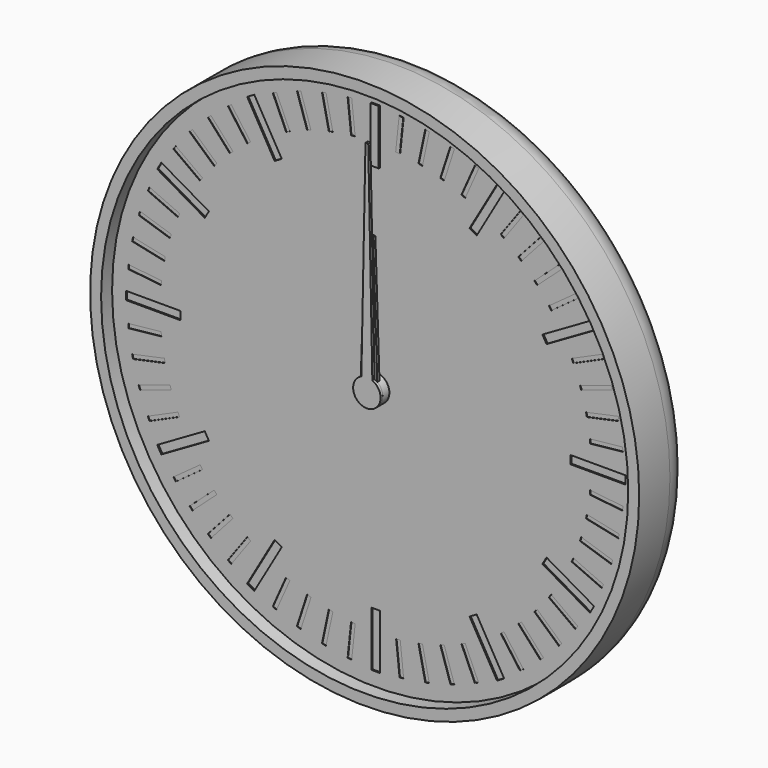
from build123d import *

# Parameters (mm, degrees)
F0_R      = 100
F1_DEPTH  = 24
F2_R      = 10
F3_T      = -4
F4_R      = 5
F4_R_2    = 3
F5_DEPTH  = 2
F6_DEPTH  = 19
F7_DEPTH  = 8
F9_DEPTH  = 4
F11_DEPTH = 4
F12_R     = 5
F12_R_2   = 3
F13_DEPTH = 2
F14_R     = 3
F15_DEPTH = 4
F17_DEPTH = 4
F18_R     = 3
F19_DEPTH = 2
F20_R     = 98
F20_R_2   = 5
F21_DEPTH = 1
F23_R     = 5
F23_R_2   = 3
F24_DEPTH = 2
F25_W     = 3
F25_H     = 20
F25_W_2   = 20
F25_H_2   = 3
F26_DEPTH = 0.5
F27_W     = 1.5
F27_H     = 12
F27_W_2   = 12
F27_H_2   = 1.5
F28_DEPTH = 0.2
F29_DEPTH = 1
F30_DEPTH = 0.4
F31_R     = 5
F31_R_2   = 3
F32_DEPTH = 5
F33_R     = 3
F34_DEPTH = 1
F36_DEPTH = 1


with BuildPart() as f1:
    # F0 (on Front) → F1 (new body)
    with BuildSketch(Plane.XZ):
        Circle(F0_R)
    extrude(amount=F1_DEPTH)

    # F2
    f2_edges = [f1.edges().sort_by_distance(p)[0] for p in [
        (-100, 0, 0),
    ]]
    fillet(f2_edges, radius=F2_R)

    # F3
    f3_openings = [f1.faces().sort_by_distance(p)[0] for p in [
        (0, -24, 0),
    ]]
    offset(amount=F3_T, openings=f3_openings)

    # F4 (on face) → F5 (join)
    with BuildSketch(Plane.XZ.offset(4)):
        Circle(F4_R)
        Circle(F4_R_2, mode=Mode.SUBTRACT)
        with Locations((40, 0)):
            Circle(F4_R)
        with Locations((40, 0)):
            Circle(F4_R_2, mode=Mode.SUBTRACT)
    extrude(amount=F5_DEPTH)


with BuildPart() as f6:
    # F6 (new): a face of the model
    f6_faces = [f1.part.faces().sort_by_distance(p)[0] for p in [
        (0, -4, 0),
    ]]
    extrude(f6_faces, amount=F6_DEPTH)

    # F8 (on face) → F9 (join)
    with BuildSketch(Plane.XZ.offset(6)):
        with BuildLine():
            ThreePointArc((9.2729637667, -1.3794085621), (9.3494561423, -0.6915886375), (9.375, 0))
            ThreePointArc((9.375, 0), (9.3494561423, 0.6915886375), (9.2729637667, 1.3794085621))
            ThreePointArc((9.2729637667, 1.3794085621), (8.9161548403, 2.8970343223), (8.3127812852, 4.3345463782))
            ThreePointArc((8.3127812852, 4.3345463782), (7.5845343223, 5.5104867402), (6.6911892658, 6.566476316))
            ThreePointArc((6.6911892658, 6.566476316), (5.5104867402, 7.5845343223), (4.1773988938, 8.3928519278))
            ThreePointArc((4.1773988938, 8.3928519278), (2.8970343223, 8.9161548403), (1.5536078905, 9.2453733036))
            ThreePointArc((1.5536078905, 9.2453733036), (0, 9.375), (-1.5536078905, 9.2453733036))
            ThreePointArc((-1.5536078905, 9.2453733036), (-2.8970343223, 8.9161548403), (-4.1773988938, 8.3928519278))
            ThreePointArc((-4.1773988938, 8.3928519278), (-5.5104867402, 7.5845343223), (-6.6911892658, 6.566476316))
            ThreePointArc((-6.6911892658, 6.566476316), (-7.5845343223, 5.5104867402), (-8.3127812852, 4.3345463782))
            ThreePointArc((-8.3127812852, 4.3345463782), (-8.9161548403, 2.8970343223), (-9.2729637667, 1.3794085621))
            ThreePointArc((-9.2729637667, 1.3794085621), (-9.375, 0), (-9.2729637667, -1.3794085621))
            ThreePointArc((-9.2729637667, -1.3794085621), (-8.9161548403, -2.8970343223), (-8.3127812852, -4.3345463782))
            ThreePointArc((-8.3127812852, -4.3345463782), (-7.5845343223, -5.5104867402), (-6.6911892658, -6.566476316))
            ThreePointArc((-6.6911892658, -6.566476316), (-5.5104867402, -7.5845343223), (-4.1773988938, -8.3928519278))
            ThreePointArc((-4.1773988938, -8.3928519278), (-2.8970343223, -8.9161548403), (-1.5536078905, -9.2453733036))
            ThreePointArc((-1.5536078905, -9.2453733036), (0, -9.375), (1.5536078905, -9.2453733036))
            ThreePointArc((1.5536078905, -9.2453733036), (2.8970343223, -8.9161548403), (4.1773988938, -8.3928519278))
            ThreePointArc((4.1773988938, -8.3928519278), (5.5104867402, -7.5845343223), (6.6911892658, -6.566476316))
            ThreePointArc((6.6911892658, -6.566476316), (7.5845343223, -5.5104867402), (8.3127812852, -4.3345463782))
            ThreePointArc((8.3127812852, -4.3345463782), (8.9161548403, -2.8970343223), (9.2729637667, -1.3794085621))
        make_face()
        with BuildLine():
            ThreePointArc((8.3127812852, 4.3345463782), (8.9161548403, 2.8970343223), (9.2729637667, 1.3794085621))
            Line((9.2729637667, 1.3794085621), (11.1823199426, 2.3946312492))
            Line((11.1823199426, 2.3946312492), (10.8182678729, 3.515068311))
            Line((10.8182678729, 3.515068311), (10.4542158031, 4.6355053728))
            Line((10.4542158031, 4.6355053728), (8.3127812852, 4.3345463782))
        make_face()
        with BuildLine():
            Line((11.1823199426, -2.3946312492), (9.2729637667, -1.3794085621))
            ThreePointArc((9.2729637667, -1.3794085621), (8.9161548403, -2.8970343223), (8.3127812852, -4.3345463782))
            Line((8.3127812852, -4.3345463782), (10.4542158031, -4.6355053728))
            Line((10.4542158031, -4.6355053728), (10.8182678729, -3.515068311))
            Line((10.8182678729, -3.515068311), (11.1823199426, -2.3946312492))
        make_face()
        with BuildLine():
            ThreePointArc((4.1773988938, 8.3928519278), (5.5104867402, 7.5845343223), (6.6911892658, 6.566476316))
            Line((6.6911892658, 6.566476316), (7.6391579371, 8.5101001246))
            Line((7.6391579371, 8.5101001246), (6.6860572448, 9.202568311))
            Line((6.6860572448, 9.202568311), (5.7329565525, 9.8950364974))
            Line((5.7329565525, 9.8950364974), (4.1773988938, 8.3928519278))
        make_face()
        with BuildLine():
            Line((7.6391579371, -8.5101001246), (6.6911892658, -6.566476316))
            ThreePointArc((6.6911892658, -6.566476316), (5.5104867402, -7.5845343223), (4.1773988938, -8.3928519278))
            Line((4.1773988938, -8.3928519278), (5.7329565525, -9.8950364974))
            Line((5.7329565525, -9.8950364974), (6.6860572448, -9.202568311))
            Line((6.6860572448, -9.202568311), (7.6391579371, -8.5101001246))
        make_face()
        with BuildLine():
            ThreePointArc((-1.5536078905, 9.2453733036), (0, 9.375), (1.5536078905, 9.2453733036))
            Line((1.5536078905, 9.2453733036), (1.1780972451, 11.375))
            Line((1.1780972451, 11.375), (0, 11.375))
            Line((0, 11.375), (-1.1780972451, 11.375))
            Line((-1.1780972451, 11.375), (-1.5536078905, 9.2453733036))
        make_face()
        with BuildLine():
            Line((1.1780972451, -11.375), (1.5536078905, -9.2453733036))
            ThreePointArc((1.5536078905, -9.2453733036), (0, -9.375), (-1.5536078905, -9.2453733036))
            Line((-1.5536078905, -9.2453733036), (-1.1780972451, -11.375))
            Line((-1.1780972451, -11.375), (0, -11.375))
            Line((0, -11.375), (1.1780972451, -11.375))
        make_face()
        with BuildLine():
            ThreePointArc((-6.6911892658, 6.566476316), (-5.5104867402, 7.5845343223), (-4.1773988938, 8.3928519278))
            Line((-4.1773988938, 8.3928519278), (-5.7329565525, 9.8950364974))
            Line((-5.7329565525, 9.8950364974), (-6.6860572448, 9.202568311))
            Line((-6.6860572448, 9.202568311), (-7.6391579371, 8.5101001246))
            Line((-7.6391579371, 8.5101001246), (-6.6911892658, 6.566476316))
        make_face()
        with BuildLine():
            Line((-5.7329565525, -9.8950364974), (-4.1773988938, -8.3928519278))
            ThreePointArc((-4.1773988938, -8.3928519278), (-5.5104867402, -7.5845343223), (-6.6911892658, -6.566476316))
            Line((-6.6911892658, -6.566476316), (-7.6391579371, -8.5101001246))
            Line((-7.6391579371, -8.5101001246), (-6.6860572448, -9.202568311))
            Line((-6.6860572448, -9.202568311), (-5.7329565525, -9.8950364974))
        make_face()
        with BuildLine():
            ThreePointArc((-9.2729637667, 1.3794085621), (-8.9161548403, 2.8970343223), (-8.3127812852, 4.3345463782))
            Line((-8.3127812852, 4.3345463782), (-10.4542158031, 4.6355053728))
            Line((-10.4542158031, 4.6355053728), (-10.8182678729, 3.515068311))
            Line((-10.8182678729, 3.515068311), (-11.1823199426, 2.3946312492))
            Line((-11.1823199426, 2.3946312492), (-9.2729637667, 1.3794085621))
        make_face()
        with BuildLine():
            Line((-10.4542158031, -4.6355053728), (-8.3127812852, -4.3345463782))
            ThreePointArc((-8.3127812852, -4.3345463782), (-8.9161548403, -2.8970343223), (-9.2729637667, -1.3794085621))
            Line((-9.2729637667, -1.3794085621), (-11.1823199426, -2.3946312492))
            Line((-11.1823199426, -2.3946312492), (-10.8182678729, -3.515068311))
            Line((-10.8182678729, -3.515068311), (-10.4542158031, -4.6355053728))
        make_face()
    extrude(amount=F9_DEPTH)

    # F35 (on face) → F36 (join)
    with BuildSketch(Plane.XZ.offset(23)):
        with BuildLine():
            ThreePointArc((-2, 4.582575695), (-2.7386127875, -4.1833001327), (5, 0))
            ThreePointArc((5, 0), (4.1833001327, 2.7386127875), (2, 4.582575695))
            ThreePointArc((2, 4.582575695), (0, 5), (-2, 4.582575695))
        make_face()
        with BuildLine():
            ThreePointArc((-2, 4.582575695), (0, 5), (2, 4.582575695))
            Line((2, 4.582575695), (0.5, 80))
            Line((0.5, 80), (0, 80))
            Line((0, 80), (-0.5, 80))
            Line((-0.5, 80), (-2, 4.582575695))
        make_face()
    extrude(amount=-F36_DEPTH)


with BuildPart() as f7:
    # F7 (new): a face of the model
    f7_faces = [f1.part.faces().sort_by_distance(p)[0] for p in [
        (40, -4, 0),
    ]]
    extrude(f7_faces, amount=F7_DEPTH)

    # F10 (on face) → F11 (join)
    with BuildSketch(Plane.XZ.offset(6)):
        with BuildLine():
            ThreePointArc((68.0829066802, -1.5381733945), (68.1144747006, -0.7693746225), (68.125, 0))
            ThreePointArc((68.125, 0), (68.1144747006, 0.7693746225), (68.0829066802, 1.5381733945))
            ThreePointArc((68.0829066802, 1.5381733945), (67.9709283072, 2.9398630294), (67.7890320221, 4.3342039956))
            ThreePointArc((67.7890320221, 4.3342039956), (67.5104012706, 5.8475163042), (67.1494235596, 7.3433252263))
            ThreePointArc((67.1494235596, 7.3433252263), (66.7484645208, 8.6911029668), (66.280643318, 10.0171558733))
            ThreePointArc((66.280643318, 10.0171558733), (65.6934659962, 11.4394680865), (65.0293803521, 12.8275385085))
            ThreePointArc((65.0293803521, 12.8275385085), (64.3569644814, 14.0625), (63.6236643925, 15.2623099717))
            ThreePointArc((63.6236643925, 15.2623099717), (62.7536029668, 16.5314602207), (61.815433119, 17.7511268046))
            ThreePointArc((61.815433119, 17.7511268046), (60.9009482166, 18.8192983038), (59.934217974, 19.8404278876))
            ThreePointArc((59.934217974, 19.8404278876), (58.8192983038, 20.9009482166), (57.6480467764, 21.8989056799))
            ThreePointArc((57.6480467764, 21.8989056799), (56.5314602207, 22.7536029668), (55.3735505752, 23.5514238999))
            ThreePointArc((55.3735505752, 23.5514238999), (54.0625, 24.3569644814), (52.709356105, 25.0895972944))
            ThreePointArc((52.709356105, 25.0895972944), (51.4394680865, 25.6934659962), (50.1409852457, 26.2331096755))
            ThreePointArc((50.1409852457, 26.2331096755), (48.6911029668, 26.7484645208), (47.2152055856, 27.1837531139))
            ThreePointArc((47.2152055856, 27.1837531139), (45.8475163042, 27.5104012706), (44.4652101991, 27.7682826779))
            ThreePointArc((44.4652101991, 27.7682826779), (42.9398630294, 27.9709283072), (41.4057159597, 28.0898484802))
            ThreePointArc((41.4057159597, 28.0898484802), (40, 28.125), (38.5942840403, 28.0898484802))
            ThreePointArc((38.5942840403, 28.0898484802), (37.0601369706, 27.9709283072), (35.5347898009, 27.7682826779))
            ThreePointArc((35.5347898009, 27.7682826779), (34.1524836958, 27.5104012706), (32.7847944144, 27.1837531139))
            ThreePointArc((32.7847944144, 27.1837531139), (31.3088970332, 26.7484645208), (29.8590147543, 26.2331096755))
            ThreePointArc((29.8590147543, 26.2331096755), (28.5605319135, 25.6934659962), (27.290643895, 25.0895972944))
            ThreePointArc((27.290643895, 25.0895972944), (25.9375, 24.3569644814), (24.6264494248, 23.5514238999))
            ThreePointArc((24.6264494248, 23.5514238999), (23.4685397793, 22.7536029668), (22.3519532236, 21.8989056799))
            ThreePointArc((22.3519532236, 21.8989056799), (21.1807016962, 20.9009482166), (20.065782026, 19.8404278876))
            ThreePointArc((20.065782026, 19.8404278876), (19.0990517834, 18.8192983038), (18.184566881, 17.7511268046))
            ThreePointArc((18.184566881, 17.7511268046), (17.2463970332, 16.5314602207), (16.3763356075, 15.2623099717))
            ThreePointArc((16.3763356075, 15.2623099717), (15.6430355186, 14.0625), (14.9706196479, 12.8275385085))
            ThreePointArc((14.9706196479, 12.8275385085), (14.3065340038, 11.4394680865), (13.719356682, 10.0171558733))
            ThreePointArc((13.719356682, 10.0171558733), (13.2515354792, 8.6911029668), (12.8505764404, 7.3433252263))
            ThreePointArc((12.8505764404, 7.3433252263), (12.4895987294, 5.8475163042), (12.2109679779, 4.3342039956))
            ThreePointArc((12.2109679779, 4.3342039956), (12.0290716928, 2.9398630294), (11.9170933198, 1.5381733945))
            ThreePointArc((11.9170933198, 1.5381733945), (11.875, 0), (11.9170933198, -1.5381733945))
            ThreePointArc((11.9170933198, -1.5381733945), (12.0290716928, -2.9398630294), (12.2109679779, -4.3342039956))
            ThreePointArc((12.2109679779, -4.3342039956), (12.4895987294, -5.8475163042), (12.8505764404, -7.3433252263))
            ThreePointArc((12.8505764404, -7.3433252263), (13.2515354792, -8.6911029668), (13.719356682, -10.0171558733))
            ThreePointArc((13.719356682, -10.0171558733), (14.3065340038, -11.4394680865), (14.9706196479, -12.8275385085))
            ThreePointArc((14.9706196479, -12.8275385085), (15.6430355186, -14.0625), (16.3763356075, -15.2623099717))
            ThreePointArc((16.3763356075, -15.2623099717), (17.2463970332, -16.5314602207), (18.184566881, -17.7511268046))
            ThreePointArc((18.184566881, -17.7511268046), (19.0990517834, -18.8192983038), (20.065782026, -19.8404278876))
            ThreePointArc((20.065782026, -19.8404278876), (21.1807016962, -20.9009482166), (22.3519532236, -21.8989056799))
            ThreePointArc((22.3519532236, -21.8989056799), (23.4685397793, -22.7536029668), (24.6264494248, -23.5514238999))
            ThreePointArc((24.6264494248, -23.5514238999), (25.9375, -24.3569644814), (27.290643895, -25.0895972944))
            ThreePointArc((27.290643895, -25.0895972944), (28.5605319135, -25.6934659962), (29.8590147543, -26.2331096755))
            ThreePointArc((29.8590147543, -26.2331096755), (31.3088970332, -26.7484645208), (32.7847944144, -27.1837531139))
            ThreePointArc((32.7847944144, -27.1837531139), (34.1524836958, -27.5104012706), (35.5347898009, -27.7682826779))
            ThreePointArc((35.5347898009, -27.7682826779), (37.0601369706, -27.9709283072), (38.5942840403, -28.0898484802))
            ThreePointArc((38.5942840403, -28.0898484802), (40, -28.125), (41.4057159597, -28.0898484802))
            ThreePointArc((41.4057159597, -28.0898484802), (42.9398630294, -27.9709283072), (44.4652101991, -27.7682826779))
            ThreePointArc((44.4652101991, -27.7682826779), (45.8475163042, -27.5104012706), (47.2152055856, -27.1837531139))
            ThreePointArc((47.2152055856, -27.1837531139), (48.6911029668, -26.7484645208), (50.1409852457, -26.2331096755))
            ThreePointArc((50.1409852457, -26.2331096755), (51.4394680865, -25.6934659962), (52.709356105, -25.0895972944))
            ThreePointArc((52.709356105, -25.0895972944), (54.0625, -24.3569644814), (55.3735505752, -23.5514238999))
            ThreePointArc((55.3735505752, -23.5514238999), (56.5314602207, -22.7536029668), (57.6480467764, -21.8989056799))
            ThreePointArc((57.6480467764, -21.8989056799), (58.8192983038, -20.9009482166), (59.934217974, -19.8404278876))
            ThreePointArc((59.934217974, -19.8404278876), (60.9009482166, -18.8192983038), (61.815433119, -17.7511268046))
            ThreePointArc((61.815433119, -17.7511268046), (62.7536029668, -16.5314602207), (63.6236643925, -15.2623099717))
            ThreePointArc((63.6236643925, -15.2623099717), (64.3569644814, -14.0625), (65.0293803521, -12.8275385085))
            ThreePointArc((65.0293803521, -12.8275385085), (65.6934659962, -11.4394680865), (66.280643318, -10.0171558733))
            ThreePointArc((66.280643318, -10.0171558733), (66.7484645208, -8.6911029668), (67.1494235596, -7.3433252263))
            ThreePointArc((67.1494235596, -7.3433252263), (67.5104012706, -5.8475163042), (67.7890320221, -4.3342039956))
            ThreePointArc((67.7890320221, -4.3342039956), (67.9709283072, -2.9398630294), (68.0829066802, -1.5381733945))
        make_face()
        with BuildLine():
            ThreePointArc((68.0829066802, 1.5381733945), (68.1144747006, 0.7693746225), (68.125, 0))
            ThreePointArc((68.125, 0), (68.1144747006, -0.7693746225), (68.0829066802, -1.5381733945))
            Line((68.0829066802, -1.5381733945), (70.125, -1.1780972451))
            Line((70.125, -1.1780972451), (70.125, 0))
            Line((70.125, 0), (70.125, 1.1780972451))
            Line((70.125, 1.1780972451), (68.0829066802, 1.5381733945))
        make_face()
        with BuildLine():
            ThreePointArc((67.1494235596, 7.3433252263), (67.5104012706, 5.8475163042), (67.7890320221, 4.3342039956))
            Line((67.7890320221, 4.3342039956), (69.7116366623, 5.1109866922))
            Line((69.7116366623, 5.1109866922), (69.4666964721, 6.2633396859))
            Line((69.4666964721, 6.2633396859), (69.2217562819, 7.4156926796))
            Line((69.2217562819, 7.4156926796), (67.1494235596, 7.3433252263))
        make_face()
        with BuildLine():
            Line((69.7116366623, -5.1109866922), (67.7890320221, -4.3342039956))
            ThreePointArc((67.7890320221, -4.3342039956), (67.5104012706, -5.8475163042), (67.1494235596, -7.3433252263))
            Line((67.1494235596, -7.3433252263), (69.2217562819, -7.4156926796))
            Line((69.2217562819, -7.4156926796), (69.4666964721, -6.2633396859))
            Line((69.4666964721, -6.2633396859), (69.7116366623, -5.1109866922))
        make_face()
        with BuildLine():
            ThreePointArc((65.0293803521, 12.8275385085), (65.6934659962, 11.4394680865), (66.280643318, 10.0171558733))
            Line((66.280643318, 10.0171558733), (67.9997322302, 11.1766959857))
            Line((67.9997322302, 11.1766959857), (67.5205569115, 12.2529413727))
            Line((67.5205569115, 12.2529413727), (67.0413815928, 13.3291867596))
            Line((67.0413815928, 13.3291867596), (65.0293803521, 12.8275385085))
        make_face()
        with BuildLine():
            Line((67.9997322302, -11.1766959857), (66.280643318, -10.0171558733))
            ThreePointArc((66.280643318, -10.0171558733), (65.6934659962, -11.4394680865), (65.0293803521, -12.8275385085))
            Line((65.0293803521, -12.8275385085), (67.0413815928, -13.3291867596))
            Line((67.0413815928, -13.3291867596), (67.5205569115, -12.2529413727))
            Line((67.5205569115, -12.2529413727), (67.9997322302, -11.1766959857))
        make_face()
        with BuildLine():
            ThreePointArc((61.815433119, 17.7511268046), (62.7536029668, 16.5314602207), (63.6236643925, 15.2623099717))
            Line((63.6236643925, 15.2623099717), (65.064105142, 16.753930033))
            Line((65.064105142, 16.753930033), (64.3716369555, 17.7070307253))
            Line((64.3716369555, 17.7070307253), (63.6791687691, 18.6601314176))
            Line((63.6791687691, 18.6601314176), (61.815433119, 17.7511268046))
        make_face()
        with BuildLine():
            Line((65.064105142, -16.753930033), (63.6236643925, -15.2623099717))
            ThreePointArc((63.6236643925, -15.2623099717), (62.7536029668, -16.5314602207), (61.815433119, -17.7511268046))
            Line((61.815433119, -17.7511268046), (63.6791687691, -18.6601314176))
            Line((63.6791687691, -18.6601314176), (64.3716369555, -17.7070307253))
            Line((64.3716369555, -17.7070307253), (65.064105142, -16.753930033))
        make_face()
        with BuildLine():
            ThreePointArc((57.6480467764, 21.8989056799), (58.8192983038, 20.9009482166), (59.934217974, 19.8404278876))
            Line((59.934217974, 19.8404278876), (61.0330563882, 21.5989369435))
            Line((61.0330563882, 21.5989369435), (60.1575595166, 22.3872378675))
            Line((60.1575595166, 22.3872378675), (59.282062645, 23.1755387915))
            Line((59.282062645, 23.1755387915), (57.6480467764, 21.8989056799))
        make_face()
        with BuildLine():
            Line((61.0330563882, -21.5989369435), (59.934217974, -19.8404278876))
            ThreePointArc((59.934217974, -19.8404278876), (58.8192983038, -20.9009482166), (57.6480467764, -21.8989056799))
            Line((57.6480467764, -21.8989056799), (59.282062645, -23.1755387915))
            Line((59.282062645, -23.1755387915), (60.1575595166, -22.3872378675))
            Line((60.1575595166, -22.3872378675), (61.0330563882, -21.5989369435))
        make_face()
        with BuildLine():
            ThreePointArc((52.709356105, 25.0895972944), (54.0625, 24.3569644814), (55.3735505752, 23.5514238999))
            Line((55.3735505752, 23.5514238999), (56.0827621424, 25.4999666665))
            Line((56.0827621424, 25.4999666665), (55.0625, 26.089015289))
            Line((55.0625, 26.089015289), (54.0422378576, 26.6780639116))
            Line((54.0422378576, 26.6780639116), (52.709356105, 25.0895972944))
        make_face()
        with BuildLine():
            Line((56.0827621424, -25.4999666665), (55.3735505752, -23.5514238999))
            ThreePointArc((55.3735505752, -23.5514238999), (54.0625, -24.3569644814), (52.709356105, -25.0895972944))
            Line((52.709356105, -25.0895972944), (54.0422378576, -26.6780639116))
            Line((54.0422378576, -26.6780639116), (55.0625, -26.089015289))
            Line((55.0625, -26.089015289), (56.0827621424, -25.4999666665))
        make_face()
        with BuildLine():
            ThreePointArc((47.2152055856, 27.1837531139), (48.6911029668, 26.7484645208), (50.1409852457, 26.2331096755))
            Line((50.1409852457, 26.2331096755), (50.4295740173, 28.2865254836))
            Line((50.4295740173, 28.2865254836), (49.3091369555, 28.6505775534))
            Line((49.3091369555, 28.6505775534), (48.1886998938, 29.0146296232))
            Line((48.1886998938, 29.0146296232), (47.2152055856, 27.1837531139))
        make_face()
        with BuildLine():
            Line((50.4295740173, -28.2865254836), (50.1409852457, -26.2331096755))
            ThreePointArc((50.1409852457, -26.2331096755), (48.6911029668, -26.7484645208), (47.2152055856, -27.1837531139))
            Line((47.2152055856, -27.1837531139), (48.1886998938, -29.0146296232))
            Line((48.1886998938, -29.0146296232), (49.3091369555, -28.6505775534))
            Line((49.3091369555, -28.6505775534), (50.4295740173, -28.2865254836))
        make_face()
        with BuildLine():
            ThreePointArc((41.4057159597, 28.0898484802), (42.9398630294, 27.9709283072), (44.4652101991, 27.7682826779))
            Line((44.4652101991, 27.7682826779), (44.3205634611, 29.8368274034))
            Line((44.3205634611, 29.8368274034), (43.1489199559, 29.959972098))
            Line((43.1489199559, 29.959972098), (41.9772764508, 30.0831167926))
            Line((41.9772764508, 30.0831167926), (41.4057159597, 28.0898484802))
        make_face()
        with BuildLine():
            Line((44.3205634611, -29.8368274034), (44.4652101991, -27.7682826779))
            ThreePointArc((44.4652101991, -27.7682826779), (42.9398630294, -27.9709283072), (41.4057159597, -28.0898484802))
            Line((41.4057159597, -28.0898484802), (41.9772764508, -30.0831167926))
            Line((41.9772764508, -30.0831167926), (43.1489199559, -29.959972098))
            Line((43.1489199559, -29.959972098), (44.3205634611, -29.8368274034))
        make_face()
        with BuildLine():
            ThreePointArc((35.5347898009, 27.7682826779), (37.0601369706, 27.9709283072), (38.5942840403, 28.0898484802))
            Line((38.5942840403, 28.0898484802), (38.0227235492, 30.0831167926))
            Line((38.0227235492, 30.0831167926), (36.8510800441, 29.959972098))
            Line((36.8510800441, 29.959972098), (35.6794365389, 29.8368274034))
            Line((35.6794365389, 29.8368274034), (35.5347898009, 27.7682826779))
        make_face()
        with BuildLine():
            Line((38.0227235492, -30.0831167926), (38.5942840403, -28.0898484802))
            ThreePointArc((38.5942840403, -28.0898484802), (37.0601369706, -27.9709283072), (35.5347898009, -27.7682826779))
            Line((35.5347898009, -27.7682826779), (35.6794365389, -29.8368274034))
            Line((35.6794365389, -29.8368274034), (36.8510800441, -29.959972098))
            Line((36.8510800441, -29.959972098), (38.0227235492, -30.0831167926))
        make_face()
        with BuildLine():
            ThreePointArc((29.8590147543, 26.2331096755), (31.3088970332, 26.7484645208), (32.7847944144, 27.1837531139))
            Line((32.7847944144, 27.1837531139), (31.8113001062, 29.0146296232))
            Line((31.8113001062, 29.0146296232), (30.6908630445, 28.6505775534))
            Line((30.6908630445, 28.6505775534), (29.5704259827, 28.2865254836))
            Line((29.5704259827, 28.2865254836), (29.8590147543, 26.2331096755))
        make_face()
        with BuildLine():
            Line((31.8113001062, -29.0146296232), (32.7847944144, -27.1837531139))
            ThreePointArc((32.7847944144, -27.1837531139), (31.3088970332, -26.7484645208), (29.8590147543, -26.2331096755))
            Line((29.8590147543, -26.2331096755), (29.5704259827, -28.2865254836))
            Line((29.5704259827, -28.2865254836), (30.6908630445, -28.6505775534))
            Line((30.6908630445, -28.6505775534), (31.8113001062, -29.0146296232))
        make_face()
        with BuildLine():
            ThreePointArc((24.6264494248, 23.5514238999), (25.9375, 24.3569644814), (27.290643895, 25.0895972944))
            Line((27.290643895, 25.0895972944), (25.9577621424, 26.6780639116))
            Line((25.9577621424, 26.6780639116), (24.9375, 26.089015289))
            Line((24.9375, 26.089015289), (23.9172378576, 25.4999666665))
            Line((23.9172378576, 25.4999666665), (24.6264494248, 23.5514238999))
        make_face()
        with BuildLine():
            Line((25.9577621424, -26.6780639116), (27.290643895, -25.0895972944))
            ThreePointArc((27.290643895, -25.0895972944), (25.9375, -24.3569644814), (24.6264494248, -23.5514238999))
            Line((24.6264494248, -23.5514238999), (23.9172378576, -25.4999666665))
            Line((23.9172378576, -25.4999666665), (24.9375, -26.089015289))
            Line((24.9375, -26.089015289), (25.9577621424, -26.6780639116))
        make_face()
        with BuildLine():
            ThreePointArc((20.065782026, 19.8404278876), (21.1807016962, 20.9009482166), (22.3519532236, 21.8989056799))
            Line((22.3519532236, 21.8989056799), (20.717937355, 23.1755387915))
            Line((20.717937355, 23.1755387915), (19.8424404834, 22.3872378675))
            Line((19.8424404834, 22.3872378675), (18.9669436118, 21.5989369435))
            Line((18.9669436118, 21.5989369435), (20.065782026, 19.8404278876))
        make_face()
        with BuildLine():
            Line((20.717937355, -23.1755387915), (22.3519532236, -21.8989056799))
            ThreePointArc((22.3519532236, -21.8989056799), (21.1807016962, -20.9009482166), (20.065782026, -19.8404278876))
            Line((20.065782026, -19.8404278876), (18.9669436118, -21.5989369435))
            Line((18.9669436118, -21.5989369435), (19.8424404834, -22.3872378675))
            Line((19.8424404834, -22.3872378675), (20.717937355, -23.1755387915))
        make_face()
        with BuildLine():
            ThreePointArc((16.3763356075, 15.2623099717), (17.2463970332, 16.5314602207), (18.184566881, 17.7511268046))
            Line((18.184566881, 17.7511268046), (16.3208312309, 18.6601314176))
            Line((16.3208312309, 18.6601314176), (15.6283630445, 17.7070307253))
            Line((15.6283630445, 17.7070307253), (14.935894858, 16.753930033))
            Line((14.935894858, 16.753930033), (16.3763356075, 15.2623099717))
        make_face()
        with BuildLine():
            Line((16.3208312309, -18.6601314176), (18.184566881, -17.7511268046))
            ThreePointArc((18.184566881, -17.7511268046), (17.2463970332, -16.5314602207), (16.3763356075, -15.2623099717))
            Line((16.3763356075, -15.2623099717), (14.935894858, -16.753930033))
            Line((14.935894858, -16.753930033), (15.6283630445, -17.7070307253))
            Line((15.6283630445, -17.7070307253), (16.3208312309, -18.6601314176))
        make_face()
        with BuildLine():
            ThreePointArc((13.719356682, 10.0171558733), (14.3065340038, 11.4394680865), (14.9706196479, 12.8275385085))
            Line((14.9706196479, 12.8275385085), (12.9586184072, 13.3291867596))
            Line((12.9586184072, 13.3291867596), (12.4794430885, 12.2529413727))
            Line((12.4794430885, 12.2529413727), (12.0002677698, 11.1766959857))
            Line((12.0002677698, 11.1766959857), (13.719356682, 10.0171558733))
        make_face()
        with BuildLine():
            Line((12.9586184072, -13.3291867596), (14.9706196479, -12.8275385085))
            ThreePointArc((14.9706196479, -12.8275385085), (14.3065340038, -11.4394680865), (13.719356682, -10.0171558733))
            Line((13.719356682, -10.0171558733), (12.0002677698, -11.1766959857))
            Line((12.0002677698, -11.1766959857), (12.4794430885, -12.2529413727))
            Line((12.4794430885, -12.2529413727), (12.9586184072, -13.3291867596))
        make_face()
        with BuildLine():
            ThreePointArc((12.2109679779, 4.3342039956), (12.4895987294, 5.8475163042), (12.8505764404, 7.3433252263))
            Line((12.8505764404, 7.3433252263), (10.7782437181, 7.4156926796))
            Line((10.7782437181, 7.4156926796), (10.5333035279, 6.2633396859))
            Line((10.5333035279, 6.2633396859), (10.2883633377, 5.1109866922))
            Line((10.2883633377, 5.1109866922), (12.2109679779, 4.3342039956))
        make_face()
        with BuildLine():
            Line((10.7782437181, -7.4156926796), (12.8505764404, -7.3433252263))
            ThreePointArc((12.8505764404, -7.3433252263), (12.4895987294, -5.8475163042), (12.2109679779, -4.3342039956))
            Line((12.2109679779, -4.3342039956), (10.2883633377, -5.1109866922))
            Line((10.2883633377, -5.1109866922), (10.5333035279, -6.2633396859))
            Line((10.5333035279, -6.2633396859), (10.7782437181, -7.4156926796))
        make_face()
        with BuildLine():
            ThreePointArc((11.9170933198, -1.5381733945), (11.875, 0), (11.9170933198, 1.5381733945))
            Line((11.9170933198, 1.5381733945), (9.875, 1.1780972451))
            Line((9.875, 1.1780972451), (9.875, 0))
            Line((9.875, 0), (9.875, -1.1780972451))
            Line((9.875, -1.1780972451), (11.9170933198, -1.5381733945))
        make_face()
    extrude(amount=F11_DEPTH)

    # F16 (on face) → F17 (join)
    with BuildSketch(Plane.XZ.offset(12)):
        with BuildLine():
            ThreePointArc((47.4288750323, -1.0304444454), (47.4821976298, -0.5164480894), (47.5, 0))
            ThreePointArc((47.5, 0), (47.4821976298, 0.5164480894), (47.4288750323, 1.0304444454))
            ThreePointArc((47.4288750323, 1.0304444454), (47.1329238722, 2.3176274578), (46.6157661985, 3.532936117))
            ThreePointArc((46.6157661985, 3.532936117), (46.0676274578, 4.4083893922), (45.4044061018, 5.2002302532))
            ThreePointArc((45.4044061018, 5.2002302532), (44.4083893922, 6.0676274578), (43.2756595386, 6.7468551628))
            ThreePointArc((43.2756595386, 6.7468551628), (42.3176274578, 7.1329238722), (41.3156377295, 7.3837048536))
            ThreePointArc((41.3156377295, 7.3837048536), (40, 7.5), (38.6843622705, 7.3837048536))
            ThreePointArc((38.6843622705, 7.3837048536), (37.6823725422, 7.1329238722), (36.7243404614, 6.7468551628))
            ThreePointArc((36.7243404614, 6.7468551628), (35.5916106078, 6.0676274578), (34.5955938982, 5.2002302532))
            ThreePointArc((34.5955938982, 5.2002302532), (33.9323725422, 4.4083893922), (33.3842338015, 3.532936117))
            ThreePointArc((33.3842338015, 3.532936117), (32.8670761278, 2.3176274578), (32.5711249677, 1.0304444454))
            ThreePointArc((32.5711249677, 1.0304444454), (32.5, 0), (32.5711249677, -1.0304444454))
            ThreePointArc((32.5711249677, -1.0304444454), (32.8670761278, -2.3176274578), (33.3842338015, -3.532936117))
            ThreePointArc((33.3842338015, -3.532936117), (33.9323725422, -4.4083893922), (34.5955938982, -5.2002302532))
            ThreePointArc((34.5955938982, -5.2002302532), (35.5916106078, -6.0676274578), (36.7243404614, -6.7468551628))
            ThreePointArc((36.7243404614, -6.7468551628), (37.6823725422, -7.1329238722), (38.6843622705, -7.3837048536))
            ThreePointArc((38.6843622705, -7.3837048536), (40, -7.5), (41.3156377295, -7.3837048536))
            ThreePointArc((41.3156377295, -7.3837048536), (42.3176274578, -7.1329238722), (43.2756595386, -6.7468551628))
            ThreePointArc((43.2756595386, -6.7468551628), (44.4083893922, -6.0676274578), (45.4044061018, -5.2002302532))
            ThreePointArc((45.4044061018, -5.2002302532), (46.0676274578, -4.4083893922), (46.6157661985, -3.532936117))
            ThreePointArc((46.6157661985, -3.532936117), (47.1329238722, -2.3176274578), (47.4288750323, -1.0304444454))
        make_face()
        with BuildLine():
            ThreePointArc((46.6157661985, 3.532936117), (47.1329238722, 2.3176274578), (47.4288750323, 1.0304444454))
            Line((47.4288750323, 1.0304444454), (49.3262785606, 2.0393117971))
            Line((49.3262785606, 2.0393117971), (48.743795249, 3.832011096))
            Line((48.743795249, 3.832011096), (46.6157661985, 3.532936117))
        make_face()
        with BuildLine():
            Line((49.3262785606, -2.0393117971), (47.4288750323, -1.0304444454))
            ThreePointArc((47.4288750323, -1.0304444454), (47.1329238722, -2.3176274578), (46.6157661985, -3.532936117))
            Line((46.6157661985, -3.532936117), (48.743795249, -3.832011096))
            Line((48.743795249, -3.832011096), (49.3262785606, -2.0393117971))
        make_face()
        with BuildLine():
            ThreePointArc((43.2756595386, 6.7468551628), (44.4083893922, 6.0676274578), (45.4044061018, 5.2002302532))
            Line((45.4044061018, 5.2002302532), (46.3464404506, 7.1316868974))
            Line((46.3464404506, 7.1316868974), (44.8214793429, 8.2396359957))
            Line((44.8214793429, 8.2396359957), (43.2756595386, 6.7468551628))
        make_face()
        with BuildLine():
            Line((46.3464404506, -7.1316868974), (45.4044061018, -5.2002302532))
            ThreePointArc((45.4044061018, -5.2002302532), (44.4083893922, -6.0676274578), (43.2756595386, -6.7468551628))
            Line((43.2756595386, -6.7468551628), (44.8214793429, -8.2396359957))
            Line((44.8214793429, -8.2396359957), (46.3464404506, -7.1316868974))
        make_face()
        with BuildLine():
            ThreePointArc((38.6843622705, 7.3837048536), (40, 7.5), (41.3156377295, 7.3837048536))
            Line((41.3156377295, 7.3837048536), (40.9424777961, 9.5))
            Line((40.9424777961, 9.5), (39.0575222039, 9.5))
            Line((39.0575222039, 9.5), (38.6843622705, 7.3837048536))
        make_face()
        with BuildLine():
            Line((40.9424777961, -9.5), (41.3156377295, -7.3837048536))
            ThreePointArc((41.3156377295, -7.3837048536), (40, -7.5), (38.6843622705, -7.3837048536))
            Line((38.6843622705, -7.3837048536), (39.0575222039, -9.5))
            Line((39.0575222039, -9.5), (40.9424777961, -9.5))
        make_face()
        with BuildLine():
            ThreePointArc((34.5955938982, 5.2002302532), (35.5916106078, 6.0676274578), (36.7243404614, 6.7468551628))
            Line((36.7243404614, 6.7468551628), (35.1785206571, 8.2396359957))
            Line((35.1785206571, 8.2396359957), (33.6535595494, 7.1316868974))
            Line((33.6535595494, 7.1316868974), (34.5955938982, 5.2002302532))
        make_face()
        with BuildLine():
            Line((35.1785206571, -8.2396359957), (36.7243404614, -6.7468551628))
            ThreePointArc((36.7243404614, -6.7468551628), (35.5916106078, -6.0676274578), (34.5955938982, -5.2002302532))
            Line((34.5955938982, -5.2002302532), (33.6535595494, -7.1316868974))
            Line((33.6535595494, -7.1316868974), (35.1785206571, -8.2396359957))
        make_face()
        with BuildLine():
            ThreePointArc((32.5711249677, 1.0304444454), (32.8670761278, 2.3176274578), (33.3842338015, 3.532936117))
            Line((33.3842338015, 3.532936117), (31.256204751, 3.832011096))
            Line((31.256204751, 3.832011096), (30.6737214394, 2.0393117971))
            Line((30.6737214394, 2.0393117971), (32.5711249677, 1.0304444454))
        make_face()
        with BuildLine():
            Line((31.256204751, -3.832011096), (33.3842338015, -3.532936117))
            ThreePointArc((33.3842338015, -3.532936117), (32.8670761278, -2.3176274578), (32.5711249677, -1.0304444454))
            Line((32.5711249677, -1.0304444454), (30.6737214394, -2.0393117971))
            Line((30.6737214394, -2.0393117971), (31.256204751, -3.832011096))
        make_face()
    extrude(amount=F17_DEPTH)

    # F18 (on face) → F19 (join)
    with BuildSketch(Plane.XZ.offset(16)):
        with Locations((40, 0)):
            Circle(F18_R)
    extrude(amount=F19_DEPTH)


with BuildPart() as f13:
    # F12 (on face) → F13 (new body)
    with BuildSketch(Plane.XZ.offset(10)):
        Circle(F12_R)
        Circle(F12_R_2, mode=Mode.SUBTRACT)
    extrude(amount=F13_DEPTH)

    # F14 (on face) → F15 (join)
    with BuildSketch(Plane.XZ.offset(12)):
        with BuildLine():
            ThreePointArc((29.9719225946, -1.2976347654), (29.9929798273, -0.6489692452), (30, 0))
            ThreePointArc((30, 0), (29.9929798273, 0.6489692452), (29.9719225946, 1.2976347654))
            ThreePointArc((29.9719225946, 1.2976347654), (29.907520012, 2.3537728718), (29.8059132922, 3.4069829492))
            ThreePointArc((29.8059132922, 3.4069829492), (29.6306502179, 4.6930339512), (29.3999236916, 5.9703004054))
            ThreePointArc((29.3999236916, 5.9703004054), (29.1710976119, 7.0033609157), (28.9059834845, 8.0277094364))
            ThreePointArc((28.9059834845, 8.0277094364), (28.5316954889, 9.2705098312), (28.1040010945, 10.4959574352))
            ThreePointArc((28.1040010945, 10.4959574352), (27.7163859753, 11.480502971), (27.2942924299, 12.4507670749))
            ThreePointArc((27.2942924299, 12.4507670749), (26.7301957257, 13.6197149922), (26.1160647186, 14.7631691588))
            ThreePointArc((26.1160647186, 14.7631691588), (25.5792049306, 15.6749569415), (25.0105253111, 16.5672455063))
            ThreePointArc((25.0105253111, 16.5672455063), (24.2705098312, 17.6335575688), (23.4850641552, 18.6668626616))
            ThreePointArc((23.4850641552, 18.6668626616), (22.812178968, 19.4834414499), (22.1109160539, 20.2757833697))
            ThreePointArc((22.1109160539, 20.2757833697), (21.2132034356, 21.2132034356), (20.2757833697, 22.1109160539))
            ThreePointArc((20.2757833697, 22.1109160539), (19.4834414499, 22.812178968), (18.6668626616, 23.4850641552))
            ThreePointArc((18.6668626616, 23.4850641552), (17.6335575688, 24.2705098312), (16.5672455063, 25.0105253111))
            ThreePointArc((16.5672455063, 25.0105253111), (15.6749569415, 25.5792049306), (14.7631691588, 26.1160647186))
            ThreePointArc((14.7631691588, 26.1160647186), (13.6197149922, 26.7301957257), (12.4507670749, 27.2942924299))
            ThreePointArc((12.4507670749, 27.2942924299), (11.480502971, 27.7163859753), (10.4959574352, 28.1040010945))
            ThreePointArc((10.4959574352, 28.1040010945), (9.2705098312, 28.5316954889), (8.0277094364, 28.9059834845))
            ThreePointArc((8.0277094364, 28.9059834845), (7.0033609157, 29.1710976119), (5.9703004054, 29.3999236916))
            ThreePointArc((5.9703004054, 29.3999236916), (4.6930339512, 29.6306502179), (3.4069829492, 29.8059132922))
            ThreePointArc((3.4069829492, 29.8059132922), (2.3537728718, 29.907520012), (1.2976347654, 29.9719225946))
            ThreePointArc((1.2976347654, 29.9719225946), (0, 30), (-1.2976347654, 29.9719225946))
            ThreePointArc((-1.2976347654, 29.9719225946), (-2.3537728718, 29.907520012), (-3.4069829492, 29.8059132922))
            ThreePointArc((-3.4069829492, 29.8059132922), (-4.6930339512, 29.6306502179), (-5.9703004054, 29.3999236916))
            ThreePointArc((-5.9703004054, 29.3999236916), (-7.0033609157, 29.1710976119), (-8.0277094364, 28.9059834845))
            ThreePointArc((-8.0277094364, 28.9059834845), (-9.2705098312, 28.5316954889), (-10.4959574352, 28.1040010945))
            ThreePointArc((-10.4959574352, 28.1040010945), (-11.480502971, 27.7163859753), (-12.4507670749, 27.2942924299))
            ThreePointArc((-12.4507670749, 27.2942924299), (-13.6197149922, 26.7301957257), (-14.7631691588, 26.1160647186))
            ThreePointArc((-14.7631691588, 26.1160647186), (-15.6749569415, 25.5792049306), (-16.5672455063, 25.0105253111))
            ThreePointArc((-16.5672455063, 25.0105253111), (-17.6335575688, 24.2705098312), (-18.6668626616, 23.4850641552))
            ThreePointArc((-18.6668626616, 23.4850641552), (-19.4834414499, 22.812178968), (-20.2757833697, 22.1109160539))
            ThreePointArc((-20.2757833697, 22.1109160539), (-21.2132034356, 21.2132034356), (-22.1109160539, 20.2757833697))
            ThreePointArc((-22.1109160539, 20.2757833697), (-22.812178968, 19.4834414499), (-23.4850641552, 18.6668626616))
            ThreePointArc((-23.4850641552, 18.6668626616), (-24.2705098312, 17.6335575688), (-25.0105253111, 16.5672455063))
            ThreePointArc((-25.0105253111, 16.5672455063), (-25.5792049306, 15.6749569415), (-26.1160647186, 14.7631691588))
            ThreePointArc((-26.1160647186, 14.7631691588), (-26.7301957257, 13.6197149922), (-27.2942924299, 12.4507670749))
            ThreePointArc((-27.2942924299, 12.4507670749), (-27.7163859753, 11.480502971), (-28.1040010945, 10.4959574352))
            ThreePointArc((-28.1040010945, 10.4959574352), (-28.5316954889, 9.2705098312), (-28.9059834845, 8.0277094364))
            ThreePointArc((-28.9059834845, 8.0277094364), (-29.1710976119, 7.0033609157), (-29.3999236916, 5.9703004054))
            ThreePointArc((-29.3999236916, 5.9703004054), (-29.6306502179, 4.6930339512), (-29.8059132922, 3.4069829492))
            ThreePointArc((-29.8059132922, 3.4069829492), (-29.907520012, 2.3537728718), (-29.9719225946, 1.2976347654))
            ThreePointArc((-29.9719225946, 1.2976347654), (-30, 0), (-29.9719225946, -1.2976347654))
            ThreePointArc((-29.9719225946, -1.2976347654), (-29.907520012, -2.3537728718), (-29.8059132922, -3.4069829492))
            ThreePointArc((-29.8059132922, -3.4069829492), (-29.6306502179, -4.6930339512), (-29.3999236916, -5.9703004054))
            ThreePointArc((-29.3999236916, -5.9703004054), (-29.1710976119, -7.0033609157), (-28.9059834845, -8.0277094364))
            ThreePointArc((-28.9059834845, -8.0277094364), (-28.5316954889, -9.2705098312), (-28.1040010945, -10.4959574352))
            ThreePointArc((-28.1040010945, -10.4959574352), (-27.7163859753, -11.480502971), (-27.2942924299, -12.4507670749))
            ThreePointArc((-27.2942924299, -12.4507670749), (-26.7301957257, -13.6197149922), (-26.1160647186, -14.7631691588))
            ThreePointArc((-26.1160647186, -14.7631691588), (-25.5792049306, -15.6749569415), (-25.0105253111, -16.5672455063))
            ThreePointArc((-25.0105253111, -16.5672455063), (-24.2705098312, -17.6335575688), (-23.4850641552, -18.6668626616))
            ThreePointArc((-23.4850641552, -18.6668626616), (-22.812178968, -19.4834414499), (-22.1109160539, -20.2757833697))
            ThreePointArc((-22.1109160539, -20.2757833697), (-21.2132034356, -21.2132034356), (-20.2757833697, -22.1109160539))
            ThreePointArc((-20.2757833697, -22.1109160539), (-19.4834414499, -22.812178968), (-18.6668626616, -23.4850641552))
            ThreePointArc((-18.6668626616, -23.4850641552), (-17.6335575688, -24.2705098312), (-16.5672455063, -25.0105253111))
            ThreePointArc((-16.5672455063, -25.0105253111), (-15.6749569415, -25.5792049306), (-14.7631691588, -26.1160647186))
            ThreePointArc((-14.7631691588, -26.1160647186), (-13.6197149922, -26.7301957257), (-12.4507670749, -27.2942924299))
            ThreePointArc((-12.4507670749, -27.2942924299), (-11.480502971, -27.7163859753), (-10.4959574352, -28.1040010945))
            ThreePointArc((-10.4959574352, -28.1040010945), (-9.2705098312, -28.5316954889), (-8.0277094364, -28.9059834845))
            ThreePointArc((-8.0277094364, -28.9059834845), (-7.0033609157, -29.1710976119), (-5.9703004054, -29.3999236916))
            ThreePointArc((-5.9703004054, -29.3999236916), (-4.6930339512, -29.6306502179), (-3.4069829492, -29.8059132922))
            ThreePointArc((-3.4069829492, -29.8059132922), (-2.3537728718, -29.907520012), (-1.2976347654, -29.9719225946))
            ThreePointArc((-1.2976347654, -29.9719225946), (0, -30), (1.2976347654, -29.9719225946))
            ThreePointArc((1.2976347654, -29.9719225946), (2.3537728718, -29.907520012), (3.4069829492, -29.8059132922))
            ThreePointArc((3.4069829492, -29.8059132922), (4.6930339512, -29.6306502179), (5.9703004054, -29.3999236916))
            ThreePointArc((5.9703004054, -29.3999236916), (7.0033609157, -29.1710976119), (8.0277094364, -28.9059834845))
            ThreePointArc((8.0277094364, -28.9059834845), (9.2705098312, -28.5316954889), (10.4959574352, -28.1040010945))
            ThreePointArc((10.4959574352, -28.1040010945), (11.480502971, -27.7163859753), (12.4507670749, -27.2942924299))
            ThreePointArc((12.4507670749, -27.2942924299), (13.6197149922, -26.7301957257), (14.7631691588, -26.1160647186))
            ThreePointArc((14.7631691588, -26.1160647186), (15.6749569415, -25.5792049306), (16.5672455063, -25.0105253111))
            ThreePointArc((16.5672455063, -25.0105253111), (17.6335575688, -24.2705098312), (18.6668626616, -23.4850641552))
            ThreePointArc((18.6668626616, -23.4850641552), (19.4834414499, -22.812178968), (20.2757833697, -22.1109160539))
            ThreePointArc((20.2757833697, -22.1109160539), (21.2132034356, -21.2132034356), (22.1109160539, -20.2757833697))
            ThreePointArc((22.1109160539, -20.2757833697), (22.812178968, -19.4834414499), (23.4850641552, -18.6668626616))
            ThreePointArc((23.4850641552, -18.6668626616), (24.2705098312, -17.6335575688), (25.0105253111, -16.5672455063))
            ThreePointArc((25.0105253111, -16.5672455063), (25.5792049306, -15.6749569415), (26.1160647186, -14.7631691588))
            ThreePointArc((26.1160647186, -14.7631691588), (26.7301957257, -13.6197149922), (27.2942924299, -12.4507670749))
            ThreePointArc((27.2942924299, -12.4507670749), (27.7163859753, -11.480502971), (28.1040010945, -10.4959574352))
            ThreePointArc((28.1040010945, -10.4959574352), (28.5316954889, -9.2705098312), (28.9059834845, -8.0277094364))
            ThreePointArc((28.9059834845, -8.0277094364), (29.1710976119, -7.0033609157), (29.3999236916, -5.9703004054))
            ThreePointArc((29.3999236916, -5.9703004054), (29.6306502179, -4.6930339512), (29.8059132922, -3.4069829492))
            ThreePointArc((29.8059132922, -3.4069829492), (29.907520012, -2.3537728718), (29.9719225946, -1.2976347654))
        make_face()
        Circle(F14_R, mode=Mode.SUBTRACT)
        with BuildLine():
            ThreePointArc((29.9719225946, 1.2976347654), (29.9929798273, 0.6489692452), (30, 0))
            ThreePointArc((30, 0), (29.9929798273, -0.6489692452), (29.9719225946, -1.2976347654))
            Line((29.9719225946, -1.2976347654), (31.9861178577, -0.9424777961))
            Line((31.9861178577, -0.9424777961), (31.9861178577, 0))
            Line((31.9861178577, 0), (31.9861178577, 0.9424777961))
            Line((31.9861178577, 0.9424777961), (29.9719225946, 1.2976347654))
        make_face()
        with BuildLine():
            ThreePointArc((29.3999236916, 5.9703004054), (29.6306502179, 4.6930339512), (29.8059132922, 3.4069829492))
            Line((29.8059132922, 3.4069829492), (31.7397516788, 4.0728569053))
            Line((31.7397516788, 4.0728569053), (31.5923156689, 5.0037312358))
            Line((31.5923156689, 5.0037312358), (31.4448796591, 5.9346055662))
            Line((31.4448796591, 5.9346055662), (29.3999236916, 5.9703004054))
        make_face()
        with BuildLine():
            Line((31.7397516788, -4.0728569053), (29.8059132922, -3.4069829492))
            ThreePointArc((29.8059132922, -3.4069829492), (29.6306502179, -4.6930339512), (29.3999236916, -5.9703004054))
            Line((29.3999236916, -5.9703004054), (31.4448796591, -5.9346055662))
            Line((31.4448796591, -5.9346055662), (31.5923156689, -5.0037312358))
            Line((31.5923156689, -5.0037312358), (31.7397516788, -4.0728569053))
        make_face()
        with BuildLine():
            ThreePointArc((28.1040010945, 10.4959574352), (28.5316954889, 9.2705098312), (28.9059834845, 8.0277094364))
            Line((28.9059834845, 8.0277094364), (30.7118474753, 8.9879043527))
            Line((30.7118474753, 8.9879043527), (30.4206058195, 9.8842540021))
            Line((30.4206058195, 9.8842540021), (30.1293641637, 10.7806036515))
            Line((30.1293641637, 10.7806036515), (28.1040010945, 10.4959574352))
        make_face()
        with BuildLine():
            Line((30.7118474753, -8.9879043527), (28.9059834845, -8.0277094364))
            ThreePointArc((28.9059834845, -8.0277094364), (28.5316954889, -9.2705098312), (28.1040010945, -10.4959574352))
            Line((28.1040010945, -10.4959574352), (30.1293641637, -10.7806036515))
            Line((30.1293641637, -10.7806036515), (30.4206058195, -9.8842540021))
            Line((30.4206058195, -9.8842540021), (30.7118474753, -8.9879043527))
        make_face()
        with BuildLine():
            ThreePointArc((26.1160647186, 14.7631691588), (26.7301957257, 13.6197149922), (27.2942924299, 12.4507670749))
            Line((27.2942924299, 12.4507670749), (28.9277156603, 13.6816397657))
            Line((28.9277156603, 13.6816397657), (28.4998396946, 14.5213936309))
            Line((28.4998396946, 14.5213936309), (28.071963729, 15.3611474961))
            Line((28.071963729, 15.3611474961), (26.1160647186, 14.7631691588))
        make_face()
        with BuildLine():
            Line((28.9277156603, -13.6816397657), (27.2942924299, -12.4507670749))
            ThreePointArc((27.2942924299, -12.4507670749), (26.7301957257, -13.6197149922), (26.1160647186, -14.7631691588))
            Line((26.1160647186, -14.7631691588), (28.071963729, -15.3611474961))
            Line((28.071963729, -15.3611474961), (28.4998396946, -14.5213936309))
            Line((28.4998396946, -14.5213936309), (28.9277156603, -13.6816397657))
        make_face()
        with BuildLine():
            ThreePointArc((23.4850641552, 18.6668626616), (24.2705098312, 17.6335575688), (25.0105253111, 16.5672455063))
            Line((25.0105253111, 16.5672455063), (26.4312874801, 18.038487801))
            Line((26.4312874801, 18.038487801), (25.8773129309, 18.8009683548))
            Line((25.8773129309, 18.8009683548), (25.3233383818, 19.5634489087))
            Line((25.3233383818, 19.5634489087), (23.4850641552, 18.6668626616))
        make_face()
        with BuildLine():
            Line((26.4312874801, -18.038487801), (25.0105253111, -16.5672455063))
            ThreePointArc((25.0105253111, -16.5672455063), (24.2705098312, -17.6335575688), (23.4850641552, -18.6668626616))
            Line((23.4850641552, -18.6668626616), (25.3233383818, -19.5634489087))
            Line((25.3233383818, -19.5634489087), (25.8773129309, -18.8009683548))
            Line((25.8773129309, -18.8009683548), (26.4312874801, -18.038487801))
        make_face()
        with BuildLine():
            ThreePointArc((20.2757833697, 22.1109160539), (21.2132034356, 21.2132034356), (22.1109160539, 20.2757833697))
            Line((22.1109160539, 20.2757833697), (23.2840332817, 21.9511684003))
            Line((23.2840332817, 21.9511684003), (22.617600841, 22.617600841))
            Line((22.617600841, 22.617600841), (21.9511684003, 23.2840332817))
            Line((21.9511684003, 23.2840332817), (20.2757833697, 22.1109160539))
        make_face()
        with BuildLine():
            Line((23.2840332817, -21.9511684003), (22.1109160539, -20.2757833697))
            ThreePointArc((22.1109160539, -20.2757833697), (21.2132034356, -21.2132034356), (20.2757833697, -22.1109160539))
            Line((20.2757833697, -22.1109160539), (21.9511684003, -23.2840332817))
            Line((21.9511684003, -23.2840332817), (22.617600841, -22.617600841))
            Line((22.617600841, -22.617600841), (23.2840332817, -21.9511684003))
        make_face()
        with BuildLine():
            ThreePointArc((16.5672455063, 25.0105253111), (17.6335575688, 24.2705098312), (18.6668626616, 23.4850641552))
            Line((18.6668626616, 23.4850641552), (19.5634489087, 25.3233383818))
            Line((19.5634489087, 25.3233383818), (18.8009683548, 25.8773129309))
            Line((18.8009683548, 25.8773129309), (18.038487801, 26.4312874801))
            Line((18.038487801, 26.4312874801), (16.5672455063, 25.0105253111))
        make_face()
        with BuildLine():
            Line((19.5634489087, -25.3233383818), (18.6668626616, -23.4850641552))
            ThreePointArc((18.6668626616, -23.4850641552), (17.6335575688, -24.2705098312), (16.5672455063, -25.0105253111))
            Line((16.5672455063, -25.0105253111), (18.038487801, -26.4312874801))
            Line((18.038487801, -26.4312874801), (18.8009683548, -25.8773129309))
            Line((18.8009683548, -25.8773129309), (19.5634489087, -25.3233383818))
        make_face()
        with BuildLine():
            ThreePointArc((12.4507670749, 27.2942924299), (13.6197149922, 26.7301957257), (14.7631691588, 26.1160647186))
            Line((14.7631691588, 26.1160647186), (15.3611474961, 28.071963729))
            Line((15.3611474961, 28.071963729), (14.5213936309, 28.4998396946))
            Line((14.5213936309, 28.4998396946), (13.6816397657, 28.9277156603))
            Line((13.6816397657, 28.9277156603), (12.4507670749, 27.2942924299))
        make_face()
        with BuildLine():
            Line((15.3611474961, -28.071963729), (14.7631691588, -26.1160647186))
            ThreePointArc((14.7631691588, -26.1160647186), (13.6197149922, -26.7301957257), (12.4507670749, -27.2942924299))
            Line((12.4507670749, -27.2942924299), (13.6816397657, -28.9277156603))
            Line((13.6816397657, -28.9277156603), (14.5213936309, -28.4998396946))
            Line((14.5213936309, -28.4998396946), (15.3611474961, -28.071963729))
        make_face()
        with BuildLine():
            ThreePointArc((8.0277094364, 28.9059834845), (9.2705098312, 28.5316954889), (10.4959574352, 28.1040010945))
            Line((10.4959574352, 28.1040010945), (10.7806036515, 30.1293641637))
            Line((10.7806036515, 30.1293641637), (9.8842540021, 30.4206058195))
            Line((9.8842540021, 30.4206058195), (8.9879043527, 30.7118474753))
            Line((8.9879043527, 30.7118474753), (8.0277094364, 28.9059834845))
        make_face()
        with BuildLine():
            Line((10.7806036515, -30.1293641637), (10.4959574352, -28.1040010945))
            ThreePointArc((10.4959574352, -28.1040010945), (9.2705098312, -28.5316954889), (8.0277094364, -28.9059834845))
            Line((8.0277094364, -28.9059834845), (8.9879043527, -30.7118474753))
            Line((8.9879043527, -30.7118474753), (9.8842540021, -30.4206058195))
            Line((9.8842540021, -30.4206058195), (10.7806036515, -30.1293641637))
        make_face()
        with BuildLine():
            ThreePointArc((3.4069829492, 29.8059132922), (4.6930339512, 29.6306502179), (5.9703004054, 29.3999236916))
            Line((5.9703004054, 29.3999236916), (5.9346055662, 31.4448796591))
            Line((5.9346055662, 31.4448796591), (5.0037312358, 31.5923156689))
            Line((5.0037312358, 31.5923156689), (4.0728569053, 31.7397516788))
            Line((4.0728569053, 31.7397516788), (3.4069829492, 29.8059132922))
        make_face()
        with BuildLine():
            Line((5.9346055662, -31.4448796591), (5.9703004054, -29.3999236916))
            ThreePointArc((5.9703004054, -29.3999236916), (4.6930339512, -29.6306502179), (3.4069829492, -29.8059132922))
            Line((3.4069829492, -29.8059132922), (4.0728569053, -31.7397516788))
            Line((4.0728569053, -31.7397516788), (5.0037312358, -31.5923156689))
            Line((5.0037312358, -31.5923156689), (5.9346055662, -31.4448796591))
        make_face()
        with BuildLine():
            ThreePointArc((-1.2976347654, 29.9719225946), (0, 30), (1.2976347654, 29.9719225946))
            Line((1.2976347654, 29.9719225946), (0.9424777961, 31.9861178577))
            Line((0.9424777961, 31.9861178577), (0, 31.9861178577))
            Line((0, 31.9861178577), (-0.9424777961, 31.9861178577))
            Line((-0.9424777961, 31.9861178577), (-1.2976347654, 29.9719225946))
        make_face()
        with BuildLine():
            Line((0.9424777961, -31.9861178577), (1.2976347654, -29.9719225946))
            ThreePointArc((1.2976347654, -29.9719225946), (0, -30), (-1.2976347654, -29.9719225946))
            Line((-1.2976347654, -29.9719225946), (-0.9424777961, -31.9861178577))
            Line((-0.9424777961, -31.9861178577), (0, -31.9861178577))
            Line((0, -31.9861178577), (0.9424777961, -31.9861178577))
        make_face()
        with BuildLine():
            ThreePointArc((-5.9703004054, 29.3999236916), (-4.6930339512, 29.6306502179), (-3.4069829492, 29.8059132922))
            Line((-3.4069829492, 29.8059132922), (-4.0728569053, 31.7397516788))
            Line((-4.0728569053, 31.7397516788), (-5.0037312358, 31.5923156689))
            Line((-5.0037312358, 31.5923156689), (-5.9346055662, 31.4448796591))
            Line((-5.9346055662, 31.4448796591), (-5.9703004054, 29.3999236916))
        make_face()
        with BuildLine():
            Line((-4.0728569053, -31.7397516788), (-3.4069829492, -29.8059132922))
            ThreePointArc((-3.4069829492, -29.8059132922), (-4.6930339512, -29.6306502179), (-5.9703004054, -29.3999236916))
            Line((-5.9703004054, -29.3999236916), (-5.9346055662, -31.4448796591))
            Line((-5.9346055662, -31.4448796591), (-5.0037312358, -31.5923156689))
            Line((-5.0037312358, -31.5923156689), (-4.0728569053, -31.7397516788))
        make_face()
        with BuildLine():
            ThreePointArc((-10.4959574352, 28.1040010945), (-9.2705098312, 28.5316954889), (-8.0277094364, 28.9059834845))
            Line((-8.0277094364, 28.9059834845), (-8.9879043527, 30.7118474753))
            Line((-8.9879043527, 30.7118474753), (-9.8842540021, 30.4206058195))
            Line((-9.8842540021, 30.4206058195), (-10.7806036515, 30.1293641637))
            Line((-10.7806036515, 30.1293641637), (-10.4959574352, 28.1040010945))
        make_face()
        with BuildLine():
            Line((-8.9879043527, -30.7118474753), (-8.0277094364, -28.9059834845))
            ThreePointArc((-8.0277094364, -28.9059834845), (-9.2705098312, -28.5316954889), (-10.4959574352, -28.1040010945))
            Line((-10.4959574352, -28.1040010945), (-10.7806036515, -30.1293641637))
            Line((-10.7806036515, -30.1293641637), (-9.8842540021, -30.4206058195))
            Line((-9.8842540021, -30.4206058195), (-8.9879043527, -30.7118474753))
        make_face()
        with BuildLine():
            ThreePointArc((-14.7631691588, 26.1160647186), (-13.6197149922, 26.7301957257), (-12.4507670749, 27.2942924299))
            Line((-12.4507670749, 27.2942924299), (-13.6816397657, 28.9277156603))
            Line((-13.6816397657, 28.9277156603), (-14.5213936309, 28.4998396946))
            Line((-14.5213936309, 28.4998396946), (-15.3611474961, 28.071963729))
            Line((-15.3611474961, 28.071963729), (-14.7631691588, 26.1160647186))
        make_face()
        with BuildLine():
            Line((-13.6816397657, -28.9277156603), (-12.4507670749, -27.2942924299))
            ThreePointArc((-12.4507670749, -27.2942924299), (-13.6197149922, -26.7301957257), (-14.7631691588, -26.1160647186))
            Line((-14.7631691588, -26.1160647186), (-15.3611474961, -28.071963729))
            Line((-15.3611474961, -28.071963729), (-14.5213936309, -28.4998396946))
            Line((-14.5213936309, -28.4998396946), (-13.6816397657, -28.9277156603))
        make_face()
        with BuildLine():
            ThreePointArc((-18.6668626616, 23.4850641552), (-17.6335575688, 24.2705098312), (-16.5672455063, 25.0105253111))
            Line((-16.5672455063, 25.0105253111), (-18.038487801, 26.4312874801))
            Line((-18.038487801, 26.4312874801), (-18.8009683548, 25.8773129309))
            Line((-18.8009683548, 25.8773129309), (-19.5634489087, 25.3233383818))
            Line((-19.5634489087, 25.3233383818), (-18.6668626616, 23.4850641552))
        make_face()
        with BuildLine():
            Line((-18.038487801, -26.4312874801), (-16.5672455063, -25.0105253111))
            ThreePointArc((-16.5672455063, -25.0105253111), (-17.6335575688, -24.2705098312), (-18.6668626616, -23.4850641552))
            Line((-18.6668626616, -23.4850641552), (-19.5634489087, -25.3233383818))
            Line((-19.5634489087, -25.3233383818), (-18.8009683548, -25.8773129309))
            Line((-18.8009683548, -25.8773129309), (-18.038487801, -26.4312874801))
        make_face()
        with BuildLine():
            ThreePointArc((-22.1109160539, 20.2757833697), (-21.2132034356, 21.2132034356), (-20.2757833697, 22.1109160539))
            Line((-20.2757833697, 22.1109160539), (-21.9511684003, 23.2840332817))
            Line((-21.9511684003, 23.2840332817), (-22.617600841, 22.617600841))
            Line((-22.617600841, 22.617600841), (-23.2840332817, 21.9511684003))
            Line((-23.2840332817, 21.9511684003), (-22.1109160539, 20.2757833697))
        make_face()
        with BuildLine():
            Line((-21.9511684003, -23.2840332817), (-20.2757833697, -22.1109160539))
            ThreePointArc((-20.2757833697, -22.1109160539), (-21.2132034356, -21.2132034356), (-22.1109160539, -20.2757833697))
            Line((-22.1109160539, -20.2757833697), (-23.2840332817, -21.9511684003))
            Line((-23.2840332817, -21.9511684003), (-22.617600841, -22.617600841))
            Line((-22.617600841, -22.617600841), (-21.9511684003, -23.2840332817))
        make_face()
        with BuildLine():
            ThreePointArc((-25.0105253111, 16.5672455063), (-24.2705098312, 17.6335575688), (-23.4850641552, 18.6668626616))
            Line((-23.4850641552, 18.6668626616), (-25.3233383818, 19.5634489087))
            Line((-25.3233383818, 19.5634489087), (-25.8773129309, 18.8009683548))
            Line((-25.8773129309, 18.8009683548), (-26.4312874801, 18.038487801))
            Line((-26.4312874801, 18.038487801), (-25.0105253111, 16.5672455063))
        make_face()
        with BuildLine():
            Line((-25.3233383818, -19.5634489087), (-23.4850641552, -18.6668626616))
            ThreePointArc((-23.4850641552, -18.6668626616), (-24.2705098312, -17.6335575688), (-25.0105253111, -16.5672455063))
            Line((-25.0105253111, -16.5672455063), (-26.4312874801, -18.038487801))
            Line((-26.4312874801, -18.038487801), (-25.8773129309, -18.8009683548))
            Line((-25.8773129309, -18.8009683548), (-25.3233383818, -19.5634489087))
        make_face()
        with BuildLine():
            ThreePointArc((-27.2942924299, 12.4507670749), (-26.7301957257, 13.6197149922), (-26.1160647186, 14.7631691588))
            Line((-26.1160647186, 14.7631691588), (-28.071963729, 15.3611474961))
            Line((-28.071963729, 15.3611474961), (-28.4998396946, 14.5213936309))
            Line((-28.4998396946, 14.5213936309), (-28.9277156603, 13.6816397657))
            Line((-28.9277156603, 13.6816397657), (-27.2942924299, 12.4507670749))
        make_face()
        with BuildLine():
            Line((-28.071963729, -15.3611474961), (-26.1160647186, -14.7631691588))
            ThreePointArc((-26.1160647186, -14.7631691588), (-26.7301957257, -13.6197149922), (-27.2942924299, -12.4507670749))
            Line((-27.2942924299, -12.4507670749), (-28.9277156603, -13.6816397657))
            Line((-28.9277156603, -13.6816397657), (-28.4998396946, -14.5213936309))
            Line((-28.4998396946, -14.5213936309), (-28.071963729, -15.3611474961))
        make_face()
        with BuildLine():
            ThreePointArc((-28.9059834845, 8.0277094364), (-28.5316954889, 9.2705098312), (-28.1040010945, 10.4959574352))
            Line((-28.1040010945, 10.4959574352), (-30.1293641637, 10.7806036515))
            Line((-30.1293641637, 10.7806036515), (-30.4206058195, 9.8842540021))
            Line((-30.4206058195, 9.8842540021), (-30.7118474753, 8.9879043527))
            Line((-30.7118474753, 8.9879043527), (-28.9059834845, 8.0277094364))
        make_face()
        with BuildLine():
            Line((-30.1293641637, -10.7806036515), (-28.1040010945, -10.4959574352))
            ThreePointArc((-28.1040010945, -10.4959574352), (-28.5316954889, -9.2705098312), (-28.9059834845, -8.0277094364))
            Line((-28.9059834845, -8.0277094364), (-30.7118474753, -8.9879043527))
            Line((-30.7118474753, -8.9879043527), (-30.4206058195, -9.8842540021))
            Line((-30.4206058195, -9.8842540021), (-30.1293641637, -10.7806036515))
        make_face()
        with BuildLine():
            ThreePointArc((-29.8059132922, 3.4069829492), (-29.6306502179, 4.6930339512), (-29.3999236916, 5.9703004054))
            Line((-29.3999236916, 5.9703004054), (-31.4448796591, 5.9346055662))
            Line((-31.4448796591, 5.9346055662), (-31.5923156689, 5.0037312358))
            Line((-31.5923156689, 5.0037312358), (-31.7397516788, 4.0728569053))
            Line((-31.7397516788, 4.0728569053), (-29.8059132922, 3.4069829492))
        make_face()
        with BuildLine():
            Line((-31.4448796591, -5.9346055662), (-29.3999236916, -5.9703004054))
            ThreePointArc((-29.3999236916, -5.9703004054), (-29.6306502179, -4.6930339512), (-29.8059132922, -3.4069829492))
            Line((-29.8059132922, -3.4069829492), (-31.7397516788, -4.0728569053))
            Line((-31.7397516788, -4.0728569053), (-31.5923156689, -5.0037312358))
            Line((-31.5923156689, -5.0037312358), (-31.4448796591, -5.9346055662))
        make_face()
        with BuildLine():
            ThreePointArc((-29.9719225946, -1.2976347654), (-30, 0), (-29.9719225946, 1.2976347654))
            Line((-29.9719225946, 1.2976347654), (-31.9861178577, 0.9424777961))
            Line((-31.9861178577, 0.9424777961), (-31.9861178577, 0))
            Line((-31.9861178577, 0), (-31.9861178577, -0.9424777961))
            Line((-31.9861178577, -0.9424777961), (-29.9719225946, -1.2976347654))
        make_face()
    extrude(amount=F15_DEPTH)

    # F31 (on face) → F32 (join)
    with BuildSketch(Plane.XZ.offset(16)):
        Circle(F31_R)
        Circle(F31_R_2, mode=Mode.SUBTRACT)
    extrude(amount=F32_DEPTH)

    # F33 (on face) → F34 (join)
    with BuildSketch(Plane.XZ.offset(21)):
        with BuildLine():
            ThreePointArc((-3, 4), (-2.2360679775, -4.472135955), (5, 0))
            ThreePointArc((5, 0), (4.472135955, 2.2360679775), (3, 4))
            ThreePointArc((3, 4), (0, 5), (-3, 4))
        make_face()
        Circle(F33_R, mode=Mode.SUBTRACT)
        with BuildLine():
            ThreePointArc((-3, 4), (0, 5), (3, 4))
            Line((3, 4), (1.5, 50))
            Line((1.5, 50), (0, 50))
            Line((0, 50), (-1.5, 50))
            Line((-1.5, 50), (-3, 4))
        make_face()
    extrude(amount=F34_DEPTH)


with BuildPart() as f21:
    # F20 (on face) → F21 (new body)
    with BuildSketch(Plane.XZ.offset(18)):
        Circle(F20_R)
        Circle(F20_R_2, mode=Mode.SUBTRACT)
    extrude(amount=F21_DEPTH)


with BuildPart() as f1_1:
    add(f1.part)

    # F22: cut F21
    add(f21.part, mode=Mode.SUBTRACT)


with BuildPart() as f21_1:
    add(f21.part)

    # F23 (on face) → F24 (join, through all)
    with BuildSketch(Plane(origin=(0, -18, 0), x_dir=(-1, 0, 0), z_dir=(0, 1, 0))):
        with Locations((-40, 0)):
            Circle(F23_R)
        with Locations((-40, 0)):
            Circle(F23_R_2, mode=Mode.SUBTRACT)
    extrude(amount=F24_DEPTH)

    # F25 (on face) → F26 (cut)
    with BuildSketch(Plane.XZ.offset(19)):
        with Locations((0, 81)):
            Rectangle(F25_W, F25_H)
        Polygon((-46.7990381057, 78.0583117444), (-36.7990381057, 60.7378036687), (-34.2009618943, 62.2378036687), (-44.2009618943, 79.5583117444), align=None)
        Polygon((-79.5583117444, 44.2009618943), (-62.2378036687, 34.2009618943), (-60.7378036687, 36.7990381057), (-78.0583117444, 46.7990381057), align=None)
        with Locations((-81, 0)):
            Rectangle(F25_W_2, F25_H_2)
        Polygon((-78.0583117444, -46.7990381057), (-60.7378036687, -36.7990381057), (-62.2378036687, -34.2009618943), (-79.5583117444, -44.2009618943), align=None)
        Polygon((-44.2009618943, -79.5583117444), (-34.2009618943, -62.2378036687), (-36.7990381057, -60.7378036687), (-46.7990381057, -78.0583117444), align=None)
        with Locations((0, -81)):
            Rectangle(F25_W, F25_H)
        Polygon((46.7990381057, -78.0583117444), (36.7990381057, -60.7378036687), (34.2009618943, -62.2378036687), (44.2009618943, -79.5583117444), align=None)
        Polygon((79.5583117444, -44.2009618943), (62.2378036687, -34.2009618943), (60.7378036687, -36.7990381057), (78.0583117444, -46.7990381057), align=None)
        with Locations((81, 0)):
            Rectangle(F25_W_2, F25_H_2)
        Polygon((78.0583117444, 46.7990381057), (60.7378036687, 36.7990381057), (62.2378036687, 34.2009618943), (79.5583117444, 44.2009618943), align=None)
        Polygon((44.2009618943, 79.5583117444), (34.2009618943, 62.2378036687), (36.7990381057, 60.7378036687), (46.7990381057, 78.0583117444), align=None)
    extrude(amount=-F26_DEPTH, mode=Mode.SUBTRACT)

    # F27 (on face) → F28 (cut)
    with BuildSketch(Plane.XZ.offset(19)):
        with Locations((0, 84.5)):
            Rectangle(F27_W, F27_H)
        Polygon((-10.2057173472, 89.9258351834), (-8.951375788, 77.991572439), (-7.459592945, 78.1483651339), (-8.7139345042, 90.0826278783), align=None)
        Polygon((-19.5496187196, 88.3664240983), (-17.0546784297, 76.6286528895), (-15.5874570286, 76.9405204257), (-18.0823973185, 88.6782916345), align=None)
        Polygon((-28.6793303782, 85.8388519789), (-24.9711264457, 74.4261737834), (-23.5445416712, 74.889699275), (-27.2527456037, 86.3023774705), align=None)
        Polygon((-37.4948252916, 82.3708114343), (-32.6139855747, 71.4082659426), (-31.2436673882, 72.0183709073), (-36.1245071051, 82.980916399), align=None)
        Polygon((-45.8995190528, 78.0002990425), (-39.8995190528, 67.6079941971), (-38.6004809472, 68.3579941971), (-44.6004809472, 78.7502990425), align=None)
        Polygon((-53.8013280783, 72.7751990517), (-46.7479050507, 63.0669951192), (-45.5343795592, 63.9486729977), (-52.5878025867, 73.6568769302), align=None)
        Polygon((-61.1136784946, 66.7527587509), (-53.0841112183, 57.8350208452), (-51.9693939801, 58.8387167547), (-59.9989612564, 67.7564546605), align=None)
        Polygon((-67.7564546605, 59.9989612564), (-58.8387167547, 51.9693939801), (-57.8350208452, 53.0841112183), (-66.7527587509, 61.1136784946), align=None)
        Polygon((-73.6568769302, 52.5878025867), (-63.9486729977, 45.5343795592), (-63.0669951192, 46.7479050507), (-72.7751990517, 53.8013280782), align=None)
        Polygon((-78.7502990425, 44.6004809472), (-68.3579941971, 38.6004809472), (-67.6079941971, 39.8995190528), (-78.0002990425, 45.8995190528), align=None)
        Polygon((-82.980916399, 36.1245071051), (-72.0183709073, 31.2436673882), (-71.4082659426, 32.6139855747), (-82.3708114343, 37.4948252916), align=None)
        Polygon((-86.3023774705, 27.2527456037), (-74.889699275, 23.5445416712), (-74.4261737834, 24.9711264457), (-85.8388519789, 28.6793303782), align=None)
        Polygon((-88.6782916345, 18.0823973185), (-76.9405204257, 15.5874570286), (-76.6286528895, 17.0546784297), (-88.3664240983, 19.5496187196), align=None)
        Polygon((-90.0826278783, 8.7139345042), (-78.1483651339, 7.459592945), (-77.991572439, 8.951375788), (-89.9258351834, 10.2057173472), align=None)
        with Locations((-84.5, 0)):
            Rectangle(F27_W_2, F27_H_2)
        Polygon((-89.9258351834, -10.2057173472), (-77.991572439, -8.951375788), (-78.1483651339, -7.459592945), (-90.0826278783, -8.7139345042), align=None)
        Polygon((-88.3664240983, -19.5496187196), (-76.6286528895, -17.0546784297), (-76.9405204257, -15.5874570286), (-88.6782916345, -18.0823973185), align=None)
        Polygon((-85.8388519789, -28.6793303782), (-74.4261737834, -24.9711264457), (-74.889699275, -23.5445416712), (-86.3023774705, -27.2527456037), align=None)
        Polygon((-82.3708114343, -37.4948252916), (-71.4082659426, -32.6139855747), (-72.0183709073, -31.2436673882), (-82.980916399, -36.1245071051), align=None)
        Polygon((-78.0002990425, -45.8995190528), (-67.6079941971, -39.8995190528), (-68.3579941971, -38.6004809472), (-78.7502990425, -44.6004809472), align=None)
        Polygon((-72.7751990517, -53.8013280783), (-63.0669951192, -46.7479050507), (-63.9486729977, -45.5343795592), (-73.6568769302, -52.5878025867), align=None)
        Polygon((-66.7527587509, -61.1136784946), (-57.8350208452, -53.0841112183), (-58.8387167547, -51.9693939801), (-67.7564546605, -59.9989612564), align=None)
        Polygon((-59.9989612564, -67.7564546605), (-51.9693939801, -58.8387167547), (-53.0841112183, -57.8350208452), (-61.1136784946, -66.7527587509), align=None)
        Polygon((-52.5878025867, -73.6568769302), (-45.5343795592, -63.9486729977), (-46.7479050507, -63.0669951192), (-53.8013280782, -72.7751990517), align=None)
        Polygon((-44.6004809472, -78.7502990425), (-38.6004809472, -68.3579941971), (-39.8995190528, -67.6079941971), (-45.8995190528, -78.0002990425), align=None)
        Polygon((-36.1245071051, -82.980916399), (-31.2436673882, -72.0183709073), (-32.6139855747, -71.4082659426), (-37.4948252916, -82.3708114343), align=None)
        Polygon((-27.2527456037, -86.3023774705), (-23.5445416712, -74.889699275), (-24.9711264457, -74.4261737834), (-28.6793303782, -85.8388519789), align=None)
        Polygon((-18.0823973185, -88.6782916345), (-15.5874570286, -76.9405204257), (-17.0546784297, -76.6286528895), (-19.5496187196, -88.3664240983), align=None)
        Polygon((-8.7139345042, -90.0826278783), (-7.459592945, -78.1483651339), (-8.951375788, -77.991572439), (-10.2057173472, -89.9258351834), align=None)
        with Locations((0, -84.5)):
            Rectangle(F27_W, F27_H)
        Polygon((10.2057173472, -89.9258351834), (8.951375788, -77.991572439), (7.459592945, -78.1483651339), (8.7139345042, -90.0826278783), align=None)
        Polygon((19.5496187196, -88.3664240983), (17.0546784297, -76.6286528895), (15.5874570286, -76.9405204257), (18.0823973185, -88.6782916345), align=None)
        Polygon((28.6793303782, -85.8388519789), (24.9711264457, -74.4261737834), (23.5445416712, -74.889699275), (27.2527456037, -86.3023774705), align=None)
        Polygon((37.4948252916, -82.3708114343), (32.6139855747, -71.4082659426), (31.2436673882, -72.0183709073), (36.1245071051, -82.980916399), align=None)
        Polygon((45.8995190528, -78.0002990425), (39.8995190528, -67.6079941971), (38.6004809472, -68.3579941971), (44.6004809472, -78.7502990425), align=None)
        Polygon((53.8013280783, -72.7751990517), (46.7479050507, -63.0669951192), (45.5343795592, -63.9486729977), (52.5878025867, -73.6568769302), align=None)
        Polygon((61.1136784946, -66.7527587509), (53.0841112183, -57.8350208452), (51.9693939801, -58.8387167547), (59.9989612564, -67.7564546605), align=None)
        Polygon((67.7564546605, -59.9989612564), (58.8387167547, -51.9693939801), (57.8350208452, -53.0841112183), (66.7527587509, -61.1136784946), align=None)
        Polygon((73.6568769302, -52.5878025867), (63.9486729977, -45.5343795592), (63.0669951192, -46.7479050507), (72.7751990517, -53.8013280782), align=None)
        Polygon((78.7502990425, -44.6004809472), (68.3579941971, -38.6004809472), (67.6079941971, -39.8995190528), (78.0002990425, -45.8995190528), align=None)
        Polygon((82.980916399, -36.1245071051), (72.0183709073, -31.2436673882), (71.4082659426, -32.6139855747), (82.3708114343, -37.4948252916), align=None)
        Polygon((86.3023774705, -27.2527456037), (74.889699275, -23.5445416712), (74.4261737834, -24.9711264457), (85.8388519789, -28.6793303782), align=None)
        Polygon((88.6782916345, -18.0823973185), (76.9405204257, -15.5874570286), (76.6286528895, -17.0546784297), (88.3664240983, -19.5496187196), align=None)
        Polygon((90.0826278783, -8.7139345042), (78.1483651339, -7.459592945), (77.991572439, -8.951375788), (89.9258351834, -10.2057173472), align=None)
        with Locations((84.5, 0)):
            Rectangle(F27_W_2, F27_H_2)
        Polygon((89.9258351834, 10.2057173472), (77.991572439, 8.951375788), (78.1483651339, 7.459592945), (90.0826278783, 8.7139345042), align=None)
        Polygon((88.3664240983, 19.5496187196), (76.6286528895, 17.0546784297), (76.9405204257, 15.5874570286), (88.6782916345, 18.0823973185), align=None)
        Polygon((85.8388519789, 28.6793303782), (74.4261737834, 24.9711264457), (74.889699275, 23.5445416712), (86.3023774705, 27.2527456037), align=None)
        Polygon((82.3708114343, 37.4948252916), (71.4082659426, 32.6139855747), (72.0183709073, 31.2436673882), (82.980916399, 36.1245071051), align=None)
        Polygon((78.0002990425, 45.8995190528), (67.6079941971, 39.8995190528), (68.3579941971, 38.6004809472), (78.7502990425, 44.6004809472), align=None)
        Polygon((72.7751990517, 53.8013280783), (63.0669951192, 46.7479050507), (63.9486729977, 45.5343795592), (73.6568769302, 52.5878025867), align=None)
        Polygon((66.7527587509, 61.1136784946), (57.8350208452, 53.0841112183), (58.8387167547, 51.9693939801), (67.7564546605, 59.9989612564), align=None)
        Polygon((59.9989612564, 67.7564546605), (51.9693939801, 58.8387167547), (53.0841112183, 57.8350208452), (61.1136784946, 66.7527587509), align=None)
        Polygon((52.5878025867, 73.6568769302), (45.5343795592, 63.9486729977), (46.7479050507, 63.0669951192), (53.8013280782, 72.7751990517), align=None)
        Polygon((44.6004809472, 78.7502990425), (38.6004809472, 68.3579941971), (39.8995190528, 67.6079941971), (45.8995190528, 78.0002990425), align=None)
        Polygon((36.1245071051, 82.980916399), (31.2436673882, 72.0183709073), (32.6139855747, 71.4082659426), (37.4948252916, 82.3708114343), align=None)
        Polygon((27.2527456037, 86.3023774705), (23.5445416712, 74.889699275), (24.9711264457, 74.4261737834), (28.6793303782, 85.8388519789), align=None)
        Polygon((18.0823973185, 88.6782916345), (15.5874570286, 76.9405204257), (17.0546784297, 76.6286528895), (19.5496187196, 88.3664240983), align=None)
        Polygon((8.7139345042, 90.0826278783), (7.459592945, 78.1483651339), (8.951375788, 77.991572439), (10.2057173472, 89.9258351834), align=None)
    extrude(amount=-F28_DEPTH, mode=Mode.SUBTRACT)


with BuildPart() as f29:
    # F29 (new): a face of the model
    f29_faces = [f21_1.part.faces().sort_by_distance(p)[0] for p in [
        (0, -18.5, 81),
    ]]
    extrude(f29_faces, amount=F29_DEPTH)


with BuildPart() as f30:
    # F30 (new): a face of the model
    f30_faces = [f21_1.part.faces().sort_by_distance(p)[0] for p in [
        (8.8326551461, -18.8, 84.0371001586),
    ]]
    extrude(f30_faces, amount=F30_DEPTH)


solid = Compound([f6.part, f7.part, f13.part, f1_1.part, f21_1.part, f29.part, f30.part])
